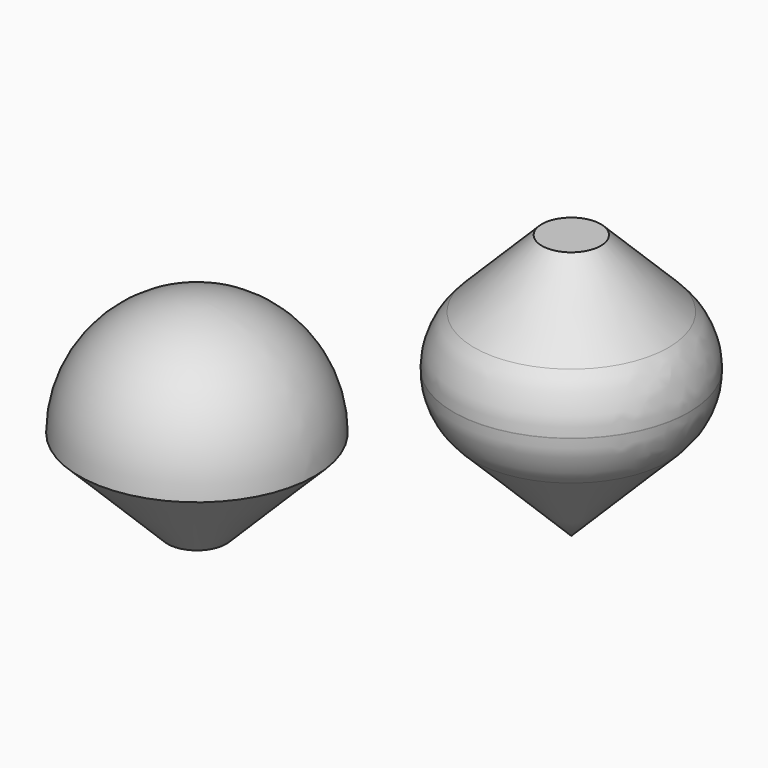
from build123d import *

# Parameters (mm, degrees)
F0_R     = 20
F1_DEPTH = 15
F2_DEPTH = 30
F3_SIZE  = 20
F4_R     = 20
F5_DEPTH = 25
F6_R     = 20
F7_DEPTH = 10
F8_SIZE  = 14.99999
F9_SIZE  = 14.99999
F10_R    = 12


# Not quite as in the source:
# - a fillet or chamfer is up to 0.001 mm smaller than in the source, because OpenCascade refuses the exact size


with BuildPart() as f1:
    # F0 (on Top) → F1 (new body)
    with BuildSketch(Plane.XY):
        with Locations((-105.1522567868, 83.3026468754)):
            Circle(F0_R)
    extrude(amount=F1_DEPTH)

    # F2 (add): a face of the model
    f2_faces = [f1.faces().sort_by_distance(p)[0] for p in [
        (-105.1522567868, 83.3026468754, 0),
    ]]
    extrude(f2_faces, amount=F2_DEPTH)

    # F3
    f3_edges = [f1.edges().sort_by_distance(p)[0] for p in [
        (-125.152257, 83.302647, -30),
    ]]
    chamfer(f3_edges, length=F3_SIZE)

    # F9 (size 15 in the source; OpenCascade refuses exactly that, so slightly less here)
    f9_edges = [f1.edges().sort_by_distance(p)[0] for p in [
        (-125.152257, 83.302647, 15),
    ]]
    chamfer(f9_edges, length=F9_SIZE)

    # F10
    f10_edges = [f1.edges().sort_by_distance(p)[0] for p in [
        (-125.152257, 83.302647, 1e-05),
        (-125.152257, 83.302647, -10),
    ]]
    fillet(f10_edges, radius=F10_R)


with BuildPart() as f5:
    # F4 (on Top) → F5 (new body)
    with BuildSketch(Plane.XY):
        with Locations((-120.4445883632, 22.9491516948)):
            Circle(F4_R)
    extrude(amount=F5_DEPTH)

    # F6
    f6_edges = [f5.edges().sort_by_distance(p)[0] for p in [
        (-140.444588, 22.949152, 25),
    ]]
    fillet(f6_edges, radius=F6_R)

    # F7 (add): a face of the model
    f7_faces = [f5.faces().sort_by_distance(p)[0] for p in [
        (-120.4445883632, 22.9491516948, 0),
    ]]
    extrude(f7_faces, amount=F7_DEPTH)

    # F8 (size 15 in the source; OpenCascade refuses exactly that, so slightly less here)
    f8_edges = [f5.edges().sort_by_distance(p)[0] for p in [
        (-140.444588, 22.949152, -10),
    ]]
    chamfer(f8_edges, length=F8_SIZE)


solid = Compound([f1.part, f5.part])
